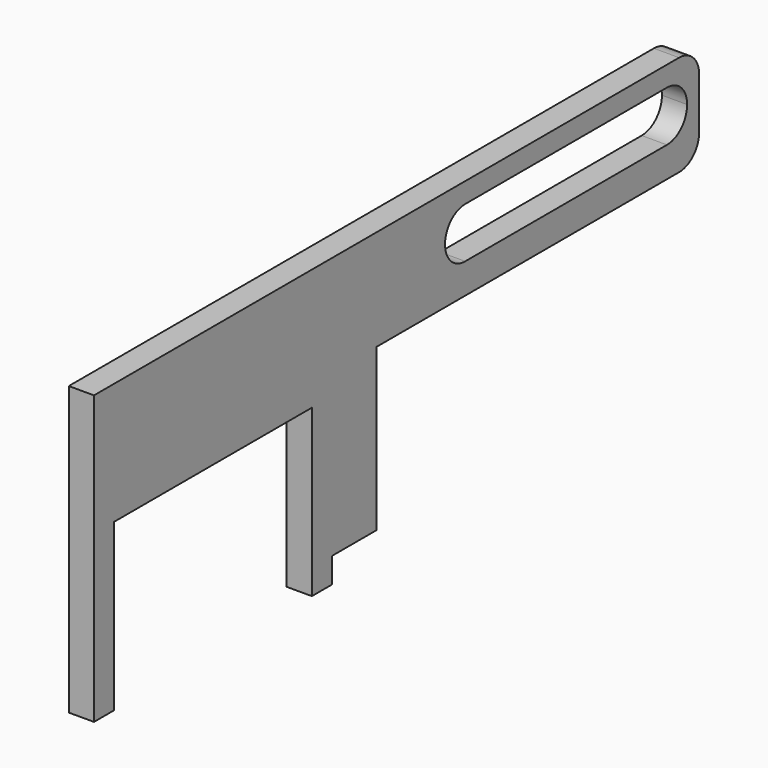
from build123d import *

# Parameters (mm, degrees)
F0_W     = 80
F0_H     = 20
F0_W_2   = 5
F0_H_2   = 5
F1_DEPTH = 5
F2_R     = 5


# Not quite as in the source:
# - a feature names something its author has since deleted; it is built from what else it names


with BuildPart() as f1:
    # F0 (on Right) → F1 (new body)
    with BuildSketch(Plane.YZ):
        with Locations((75, 42)):
            Rectangle(F0_W, F0_H)
        with BuildLine():
            ThreePointArc((107, 48), (110.5355339059, 46.5355339059), (112, 43))
            ThreePointArc((112, 43), (110.5355339059, 39.4644660941), (107, 38))
            Line((107, 38), (57, 38))
            ThreePointArc((57, 38), (52, 43), (57, 48))
            Line((57, 48), (107, 48))
        make_face(mode=Mode.SUBTRACT)
        Polygon((35, 52), (-35, 52), (-35, 0), (-30, 0), (-30, 27.9), (19, 27.9), (19, 0), (24, 0), (35, 0), (35, 32), align=None)
        with Locations((21.5, -2.5)):
            Rectangle(F0_W_2, F0_H_2)
        with Locations((-32.5, -2.5)):
            Rectangle(F0_W_2, F0_H_2)
    extrude(amount=F1_DEPTH)

    # F2
    f2_edges = [f1.edges().sort_by_distance(p)[0] for p in [
        (2.5, 115, 52),
        (2.5, 115, 32),
    ]]
    fillet(f2_edges, radius=F2_R)


solid = f1.part
